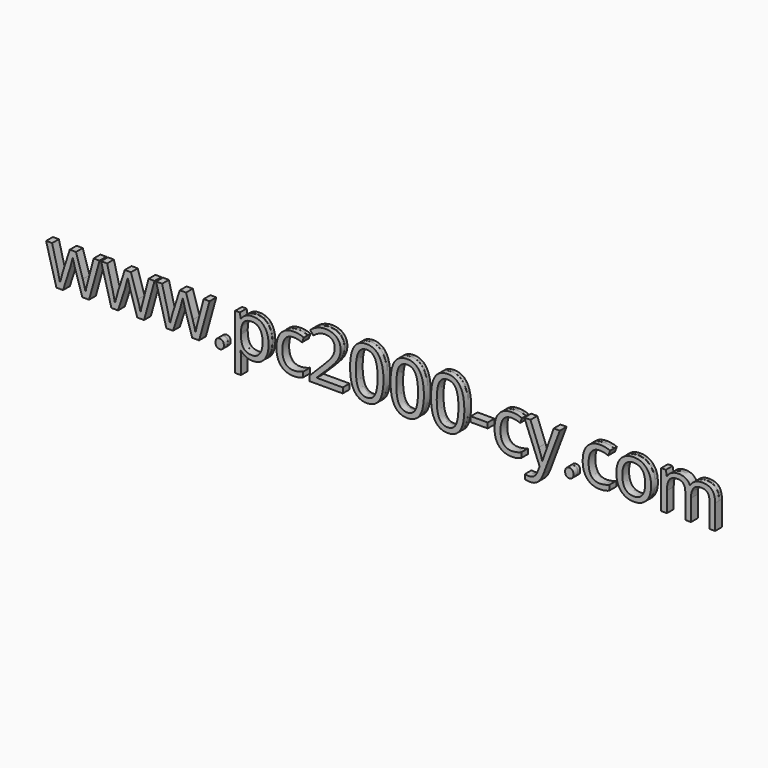
from build123d import *

# Parameters (mm, degrees)
F0_TEXT_SIZE = 208.3333333333
F1_DEPTH     = 10
F2_DEPTH     = 25
F3_DEPTH     = 25


# Not quite as in the source:
# - Text() gives the source's letters only with a copy of the font that has no kerning and outlines rounded to 1/6400 em; it was checked with that copy


with BuildPart() as f1:
    # F0 (on Front) → F1 (new body)
    with BuildSketch(Plane.XZ):
        with Locations((-352.0231353683, 13.4393077636)):
            Text('www.pc2000-cy.com', F0_TEXT_SIZE, font='Open Sans', text_align=(TextAlign.LEFT, TextAlign.BOTTOM))
    extrude(amount=F1_DEPTH)


with BuildPart() as f2:
    # F0 (on Front) → F2 (new body)
    with BuildSketch(Plane.XZ):
        with Locations((-352.0231353683, 13.4393077636)):
            Text('www.pc2000-cy.com', F0_TEXT_SIZE, font='Open Sans', text_align=(TextAlign.LEFT, TextAlign.BOTTOM))
    extrude(amount=F2_DEPTH)


with BuildPart() as f3:
    # F0 (on Front) → F3 (new body)
    with BuildSketch(Plane.XZ):
        with Locations((-352.0231353683, 13.4393077636)):
            Text('www.pc2000-cy.com', F0_TEXT_SIZE, font='Open Sans', text_align=(TextAlign.LEFT, TextAlign.BOTTOM))
    extrude(amount=F3_DEPTH)


solid = Compound([f1.part, f2.part, f3.part])
